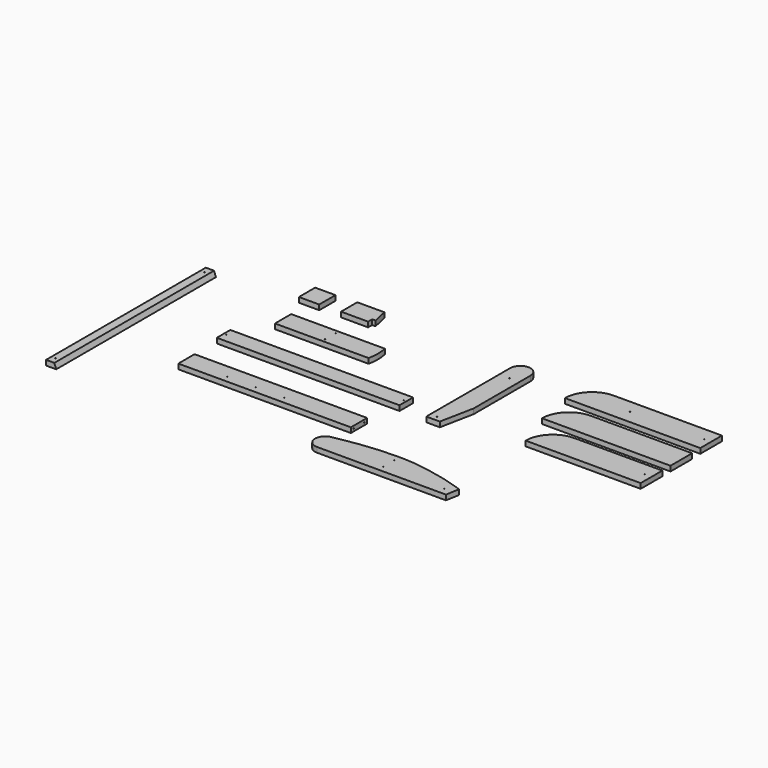
from build123d import *

# Parameters (mm, degrees)
F0_R      = 1.27
F1_DEPTH  = 19.05
F4_R      = 1.27
F5_DEPTH  = 19.05
F6_R      = 1.27
F7_DEPTH  = 19.05
F8_R      = 1.27
F9_DEPTH  = 19.05
F10_R     = 1.27
F11_DEPTH = 19.05
F12_R     = 1.27
F13_DEPTH = 19.05
F15_DEPTH = 749.3
F16_R     = 1.27
F17_DEPTH = 19.05
F18_R     = 1.27
F19_DEPTH = 19.05
F20_W     = 76.2
F20_H     = 76.2
F21_DEPTH = 19.05
F23_DEPTH = 19.05
F28_DEPTH = 19.05
F29_R     = 1.27
F30_DEPTH = 19.05
F31_R     = 1.27
F32_DEPTH = 19.05
F33_R     = 1.27
F34_DEPTH = 19.05


# Not quite as in the source:
# - the program builds the solid bodies; features that only make, move or delete a surface that nothing else refers to are left out


with BuildPart() as f1:
    # F0 (on Top) → F1 (new body)
    with BuildSketch(Plane.XY):
        with BuildLine():
            Line((-60.932392, 59.310776), (-60.932392, -334.389224))
            Line((-60.932392, -334.389224), (-10.132392, -334.389224))
            Line((-10.132392, -334.389224), (15.267608, -207.389224))
            Line((15.267608, -207.389224), (15.267608, 59.310776))
            ThreePointArc((15.267608, 59.310776), (4.108376, 86.251544), (-22.832392, 97.410776))
            ThreePointArc((-22.832392, 97.410776), (-49.773161, 86.251544), (-60.932392, 59.310776))
        make_face()
        with Locations((-35.532392, -315.339224)):
            Circle(F0_R, mode=Mode.SUBTRACT)
        with BuildLine():
            ThreePointArc((-22.832392, 9.780776), (-21.934367, 9.408801), (-21.562392, 8.510776))
            ThreePointArc((-21.562392, 8.510776), (-23.730418, 7.61275), (-22.832392, 9.780776))
        make_face(mode=Mode.SUBTRACT)
    extrude(amount=F1_DEPTH)


with BuildPart() as f2_1:
    # F2: copy of F1
    add(f1.part.moved(Location((812.8, 0, 0))))


with BuildPart() as f5:
    # F4 (on Top) → F5 (new body)
    with BuildSketch(Plane.XY):
        with BuildLine():
            ThreePointArc((363.472351, -170.081087), (291.630302, -199.839038), (261.872351, -271.681087))
            Line((261.872351, -271.681087), (693.672351, -271.681087))
            Line((693.672351, -271.681087), (693.672351, -220.881087))
            Line((693.672351, -220.881087), (693.672351, -170.081087))
            Line((693.672351, -170.081087), (363.472351, -170.081087))
        make_face()
        with Locations((668.272351, -220.881087)):
            Circle(F4_R, mode=Mode.SUBTRACT)
    extrude(amount=F5_DEPTH)


with BuildPart() as f7:
    # F6 (on Top) → F7 (new body)
    with BuildSketch(Plane.XY):
        with BuildLine():
            Line((210.500181, -131.009649), (693.100181, -131.009649))
            Line((693.100181, -131.009649), (693.100181, -80.209649))
            Line((693.100181, -80.209649), (693.100181, -29.409649))
            Line((693.100181, -29.409649), (312.100181, -29.409649))
            ThreePointArc((312.100181, -29.409649), (240.258132, -59.167601), (210.500181, -131.009649))
        make_face()
        with Locations((667.700181, -80.209649)):
            Circle(F6_R, mode=Mode.SUBTRACT)
    extrude(amount=F7_DEPTH)


with BuildPart() as f9:
    # F8 (on Top) → F9 (new body)
    with BuildSketch(Plane.XY):
        with BuildLine():
            Line((183.11931, 11.164315), (691.11931, 11.164315))
            Line((691.11931, 11.164315), (691.11931, 61.964315))
            Line((691.11931, 61.964315), (691.11931, 112.764315))
            Line((691.11931, 112.764315), (284.71931, 112.764315))
            ThreePointArc((284.71931, 112.764315), (212.877261, 83.006364), (183.11931, 11.164315))
        make_face()
        with Locations((386.31931, 61.964315)):
            Circle(F8_R, mode=Mode.SUBTRACT)
        with Locations((665.71931, 61.964315)):
            Circle(F8_R, mode=Mode.SUBTRACT)
    extrude(amount=F9_DEPTH)


with BuildPart() as f11:
    # F10 (on Top) → F11 (new body)
    with BuildSketch(Plane.XY):
        with BuildLine():
            ThreePointArc((-192.656518, -609.057055), (-228.063516, -648.512913), (-189.759585, -685.163002))
            Line((-189.759585, -685.163002), (39.529742, -685.163002))
            Line((39.529742, -685.163002), (39.529742, -662.13299))
            ThreePointArc((39.529742, -662.13299), (38.259742, -660.86299), (39.529742, -659.59299))
            Line((39.529742, -659.59299), (39.529742, -611.33299))
            ThreePointArc((39.529742, -611.33299), (38.259742, -610.06299), (39.529742, -608.79299))
            Line((39.529742, -608.79299), (39.529742, -584.66299))
            add(Edge.make_bspline(
                [(39.529742, -584.66299), (8.240435, -584.48981), (-69.693829, -586.989314), (-164.102703, -603.394447), (-192.656518, -609.057055)],
                knots=[0.566257, 0.566257, 0.566257, 0.566257, 0.77812, 1, 1, 1, 1], degree=3))
        make_face()
        with BuildLine():
            Line((39.529742, -662.13299), (39.529742, -685.163002))
            Line((39.529742, -685.163002), (293.529742, -685.163002))
            Line((293.529742, -685.163002), (302.649135, -634.363002))
            add(Edge.make_bspline(
                [(302.649135, -634.363002), (272.109092, -624.904008), (239.994661, -612.093395), (113.364797, -587.287349), (65.492526, -584.806689), (39.529742, -584.66299)],
                knots=[0.000416, 0.000416, 0.000416, 0.000416, 0.171079, 0.390461, 0.566257, 0.566257, 0.566257, 0.566257], degree=3))
            Line((39.529742, -584.66299), (39.529742, -608.79299))
            ThreePointArc((39.529742, -608.79299), (40.427768, -609.164964), (40.799742, -610.06299))
            ThreePointArc((40.799742, -610.06299), (40.427768, -610.961016), (39.529742, -611.33299))
            Line((39.529742, -611.33299), (39.529742, -659.59299))
            ThreePointArc((39.529742, -659.59299), (40.427768, -659.964964), (40.799742, -660.86299))
            ThreePointArc((40.799742, -660.86299), (40.427768, -661.761016), (39.529742, -662.13299))
        make_face()
        with Locations((267.440415, -659.763002)):
            Circle(F10_R, mode=Mode.SUBTRACT)
    extrude(amount=F11_DEPTH)


with BuildPart() as f13:
    # F12 (on Top) → F13 (new body)
    with BuildSketch(Plane.XY):
        Polygon((-838.564605, -500.333173), (-838.564605, -525.733173), (-190.864605, -525.733173), (-190.864605, -449.533173), (-838.564605, -449.533173), align=None)
        with Locations((-781.414605, -500.333173)):
            Circle(F12_R, mode=Mode.SUBTRACT)
        with Locations((-674.734605, -500.333173)):
            Circle(F12_R, mode=Mode.SUBTRACT)
        with Locations((-568.054605, -500.333173)):
            Circle(F12_R, mode=Mode.SUBTRACT)
        with Locations((-461.374605, -500.333173)):
            Circle(F12_R, mode=Mode.SUBTRACT)
        with Locations((-354.694605, -500.333173)):
            Circle(F12_R, mode=Mode.SUBTRACT)
        with Locations((-248.014605, -500.333173)):
            Circle(F12_R, mode=Mode.SUBTRACT)
    extrude(amount=F13_DEPTH)

    # F29 (on face) → F30 (cut)
    with BuildSketch(Plane(origin=(-838.564605, 0, 0), x_dir=(0, -1, 0), z_dir=(-1, 0, 0))):
        with Locations((462.233173, 9.525)):
            Circle(F29_R)
        with Locations((513.033173, 9.525)):
            Circle(F29_R)
    extrude(amount=-F30_DEPTH, mode=Mode.SUBTRACT)

    # F31 (on face) → F32 (cut)
    with BuildSketch(Plane.YZ.offset(-190.864605)):
        with Locations((-462.233173, 9.525)):
            Circle(F31_R)
        with BuildLine():
            ThreePointArc((-514.303173, 9.525), (-513.033173, 8.255), (-511.763173, 9.525))
            ThreePointArc((-511.763173, 9.525), (-513.033173, 10.795), (-514.303173, 9.525))
        make_face()
    extrude(amount=-F32_DEPTH, mode=Mode.SUBTRACT)


with BuildPart() as f15:
    # F14 (on Front) → F15 (new body)
    with BuildSketch(Plane.XZ):
        Polygon((-1156.008205, 19.05), (-1156.008205, 0), (-1117.908205, 0), (-1125.008583, 19.05), align=None)
    extrude(amount=F15_DEPTH)

    # F27 (on face) → F28 (cut)
    with BuildSketch(Plane.XY.offset(19.05)):
        with BuildLine():
            ThreePointArc((-1140.508394, -725.17), (-1139.610369, -724.798026), (-1139.238394, -723.9))
            ThreePointArc((-1139.238394, -723.9), (-1141.40642, -723.001974), (-1140.508394, -725.17))
        make_face()
        with BuildLine():
            ThreePointArc((-1140.508394, -24.13), (-1141.40642, -26.298026), (-1139.238394, -25.4))
            ThreePointArc((-1139.238394, -25.4), (-1139.610369, -24.501974), (-1140.508394, -24.13))
        make_face()
    extrude(amount=-F28_DEPTH, mode=Mode.SUBTRACT)


with BuildPart() as f17:
    # F16 (on Top) → F17 (new body)
    with BuildSketch(Plane.XY):
        Polygon((-852.784672, -263.863193), (-852.784672, -327.363193), (-166.984672, -327.363193), (-166.984672, -295.613193), (-166.984672, -263.863193), align=None)
        with Locations((-843.005672, -295.613193)):
            Circle(F16_R, mode=Mode.SUBTRACT)
        with Locations((-176.255672, -295.613193)):
            Circle(F16_R, mode=Mode.SUBTRACT)
    extrude(amount=F17_DEPTH)

    # F33 (on face) → F34 (cut)
    with BuildSketch(Plane(origin=(-852.784672, 0, 0), x_dir=(0, -1, 0), z_dir=(-1, 0, 0))):
        with Locations((295.613193, 9.525)):
            Circle(F33_R)
    extrude(amount=-F34_DEPTH, mode=Mode.SUBTRACT)


with BuildPart() as f19:
    # F18 (on Top) → F19 (new body)
    with BuildSketch(Plane.XY):
        with BuildLine():
            Line((-424.947367, -73.803925), (-776.417255, -73.803925))
            Line((-776.417255, -73.803925), (-776.417255, -150.003925))
            Line((-776.417255, -150.003925), (-598.617255, -150.003925))
            Line((-598.617255, -150.003925), (-424.947367, -150.003925))
            ThreePointArc((-424.947367, -150.003925), (-420.817255, -111.903925), (-424.947367, -73.803925))
        make_face()
        with BuildLine():
            ThreePointArc((-597.347255, -137.303925), (-597.71923, -138.201951), (-598.617255, -138.573925))
            ThreePointArc((-598.617255, -138.573925), (-599.515281, -136.405899), (-597.347255, -137.303925))
        make_face(mode=Mode.SUBTRACT)
        with Locations((-598.617255, -86.503925)):
            Circle(F18_R, mode=Mode.SUBTRACT)
    extrude(amount=F19_DEPTH)


with BuildPart() as f21:
    # F20 (on Top) → F21 (new body)
    with BuildSketch(Plane.XY):
        with Locations((-788.341646, 63.181495)):
            Rectangle(F20_W, F20_H)
    extrude(amount=F21_DEPTH)


with BuildPart() as f23:
    # F22 (on Top) → F23 (new body)
    with BuildSketch(Plane.XY):
        Polygon((-570.377707, 105.829176), (-671.977707, 105.829176), (-671.977707, 29.629176), (-570.377707, 29.629176), (-570.377707, 48.679176), (-557.677707, 48.679176), align=None)
    extrude(amount=F23_DEPTH)


solid = Compound([f1.part, f5.part, f7.part, f9.part, f11.part, f13.part, f15.part, f17.part, f19.part, f21.part, f23.part])
